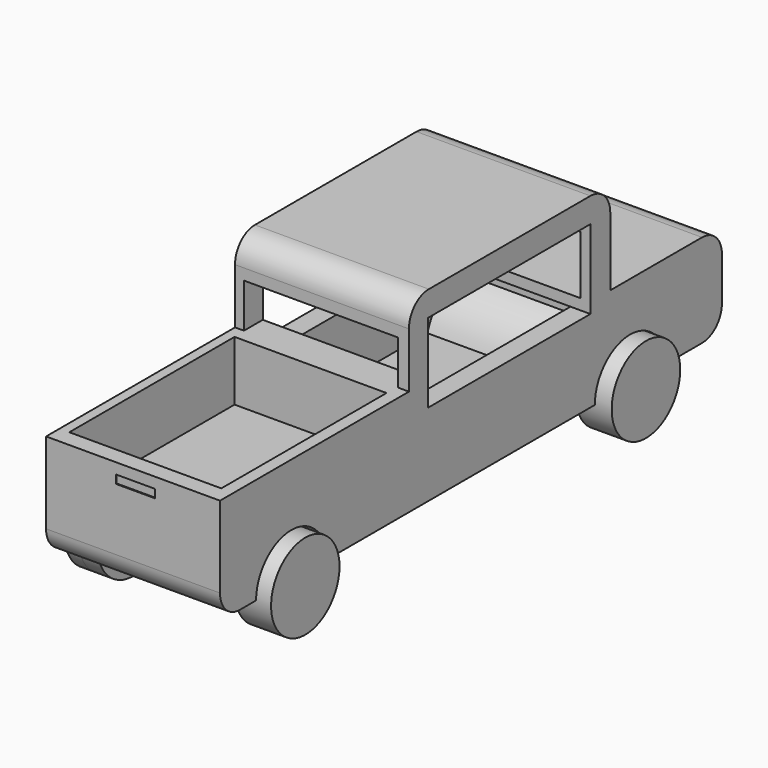
from build123d import *

# Parameters (mm, degrees)
F1_DEPTH      = 44.45
F3_DEPTH      = 46.99
F4_W          = 38.835483836
F4_H          = 52.7764223516
F5_DEPTH      = 15.24
F7_START      = 39.116
F6_R          = 10.9261370184
F7_DEPTH      = 9.144
F6_R_2        = 10.9431249162
F8_R          = 11.010831959
F9_DEPTH      = 3.556
F9_DEPTH_BACK = 4.826
F8_R_2        = 11.5864067576
F10_W         = 10.0583992898
F10_H         = 2.1336004138
F11_DEPTH     = 0.254
F12_W         = 51.9430035889
F12_H         = 20.2183979881
F13_DEPTH     = 55.118
F14_W         = 39.3191990443
F14_H         = 11.2776011229
F15_DEPTH     = 25.4
F16_T         = 5.08
F16_T3_DEPTH  = 54.61
F16_T5_DEPTH  = 12.4460015742
F16_T7_DEPTH  = 13.0047993815
F16_T9_DEPTH  = 16.1797990388
F16_T11_DEPTH = 25.4
F16_T13_DEPTH = 62.9364223516
F16_T15_DEPTH = 48.995483836
F16_T17_DEPTH = 10.414
F16_T19_DEPTH = 12.2936004138
F16_T21_DEPTH = 20.2183992898
F17_W         = 39.0143997502
F17_H         = 14.9351991713
F18_DEPTH     = 25.4


# Not quite as in the source:
# - a shell that OpenCascade refuses in one call is made with other operations: the cavity is built on its own and cut out


with BuildPart() as f1:
    # F0 (on Right) → F1 (new body)
    with BuildSketch(Plane.YZ):
        with BuildLine():
            Line((34.8995998502, 0), (34.8995998502, 23.7744003534))
            Line((34.8995998502, 23.7744003534), (34.8995998502, 41.2495988739))
            ThreePointArc((34.8995998502, 41.2495988739), (33.0397279107, 45.7397269344), (28.5495998502, 47.5995988739))
            Line((28.5495998502, 47.5995988739), (-23.0632027775, 47.5995988739))
            ThreePointArc((-23.0632027775, 47.5995988739), (-27.553330838, 45.7397269344), (-29.4132027775, 41.2495988739))
            Line((-29.4132027775, 41.2495988739), (-29.4132027775, 27.127198875))
            Line((-29.4132027775, 27.127198875), (-29.4132027775, 0))
            Line((-29.4132027775, 0), (34.8995998502, 0))
        make_face()
        with BuildLine():
            Line((-83.4136041045, 0), (-29.4132027775, 0))
            Line((-29.4132027775, 0), (-29.4132027775, 27.127198875))
            Line((-29.4132027775, 27.127198875), (-89.7636041045, 27.127198875))
            Line((-89.7636041045, 27.127198875), (-89.7636041045, 6.35))
            ThreePointArc((-89.7636041045, 6.35), (-87.9037321651, 1.8598719395), (-83.4136041045, 0))
        make_face()
        with BuildLine():
            Line((64.2112003803, 23.7744003534), (34.8995998502, 23.7744003534))
            Line((34.8995998502, 23.7744003534), (34.8995998502, 0))
            Line((34.8995998502, 0), (64.2112003803, 0))
            ThreePointArc((64.2112003803, 0), (68.7013284409, 1.8598719395), (70.5612003803, 6.35))
            Line((70.5612003803, 6.35), (70.5612003803, 17.4244003534))
            ThreePointArc((70.5612003803, 17.4244003534), (68.7013284409, 21.914528414), (64.2112003803, 23.7744003534))
        make_face()
    extrude(amount=F1_DEPTH)

    # F2 (on face) → F3 (cut)
    with BuildSketch(Plane.YZ.offset(44.45)):
        with BuildLine():
            ThreePointArc((52.4891002785, 0), (41.2242002785, 11.2649), (29.9593002785, 0))
            Line((29.9593002785, 0), (52.4891002785, 0))
        make_face()
        with BuildLine():
            Line((-78.2477574524, 0), (-55.7118488375, 0))
            ThreePointArc((-55.7118488375, 0), (-66.9798031449, 11.2679543074), (-78.2477574524, 0))
        make_face()
        with BuildLine():
            Line((52.4891002785, 0), (29.9593002785, 0))
            ThreePointArc((29.9593002785, 0), (41.2242002785, -11.2649), (52.4891002785, 0))
        make_face()
        with BuildLine():
            ThreePointArc((-78.2477574524, 0), (-66.9798031449, -11.2679543074), (-55.7118488375, 0))
            Line((-55.7118488375, 0), (-78.2477574524, 0))
        make_face()
    extrude(amount=-F3_DEPTH, mode=Mode.SUBTRACT)

    # F4 (on face) → F5 (cut)
    with BuildSketch(Plane.XY.offset(27.127198875)):
        with Locations((21.9071976608, -59.0603370219)):
            Rectangle(F4_W, F4_H)
    extrude(amount=-F5_DEPTH, mode=Mode.SUBTRACT)

    # F10 (on face) → F11 (cut)
    with BuildSketch(Plane.XZ.offset(89.7636041045)):
        with Locations((22.85999991, 23.317201063)):
            Rectangle(F10_W, F10_H)
    extrude(amount=-F11_DEPTH, mode=Mode.SUBTRACT)

    # F12 (on face) → F13 (cut)
    with BuildSketch(Plane(origin=(0, 0, 0), x_dir=(0, -1, 0), z_dir=(-1, 0, 0))):
        with Locations((-2.5780980557, 31.1403998798)):
            Rectangle(F12_W, F12_H)
    extrude(amount=-F13_DEPTH, mode=Mode.SUBTRACT)

    # F14 (on face) → F15 (cut)
    with BuildSketch(Plane.XZ.offset(29.4132027775)):
        with Locations((21.9456010964, 32.7659994364)):
            Rectangle(F14_W, F14_H)
    extrude(amount=-F15_DEPTH, mode=Mode.SUBTRACT)

    # F16: shell of thickness 5.08, made by hand


with BuildPart() as f7:
    # F6 (on Right) → F7 (new body)
    with BuildSketch(Plane.YZ.offset(F7_START)):
        with Locations((-67.2845989466, 0)):
            Circle(F6_R)
    extrude(amount=F7_DEPTH)


with BuildPart() as f7b:
    # F6 (on Right) → F7, piece 2 (new body)
    with BuildSketch(Plane.YZ.offset(F7_START)):
        with Locations((41.5289998055, 0)):
            Circle(F6_R_2)
    extrude(amount=F7_DEPTH)


with BuildPart() as f9:
    # F8 (on Right) → F9 (new body, two sides)
    with BuildSketch(Plane.YZ) as f9_sk:
        with Locations((41.8337993324, 0)):
            Circle(F8_R)
    extrude(amount=-F9_DEPTH)
    extrude(f9_sk.sketch, amount=F9_DEPTH_BACK)


with BuildPart() as f9b:
    # F8 (on Right) → F9, piece 2 (new body, two sides)
    with BuildSketch(Plane.YZ) as f9_2_sk:
        with Locations((-67.8941980004, 0)):
            Circle(F8_R_2)
    extrude(amount=-F9_DEPTH)
    extrude(f9_2_sk.sketch, amount=F9_DEPTH_BACK)


with BuildPart() as f16_core1:
    # F16_t2: copy of F1
    add(f1.part)

    # the walls: a layer under each face that stays
    f16_faces = [f16_core1.faces().sort_by_distance(p)[0] for p in [
        (22.225, 34.8995998502, 32.5119996136),
        (22.225, 49.5554001153, 23.7744003534),
        (22.225, 33.0397279107, 45.7397269344),
        (0, -63.042803357, 23.7997994369),
        (44.45, -63.042803357, 23.7997994369),
        (22.225, 68.7013284409, 21.914528414),
        (22.225, 2.7431985363, 47.5995988739),
        (22.225, 70.5612003803, 11.8872001767),
        (22.225, 68.7013284409, 1.8598719395),
        (22.225, 58.3501503294, 0),
        (22.225, -27.553330838, 45.7397269344),
        (22.225, 41.2242002785, 11.2649),
        (37.0416666667, -29.4132027775, 38.8958655407),
        (22.225, -12.8762742795, 0),
        (41.275, -28.1341323363, 27.127198875),
        (22.225, -66.9798031449, 11.2679543074),
        (22.225, -89.7636041045, 16.7385994375),
        (22.225, -80.8306807784, 0),
        (22.225, -87.9037321651, 1.8598719395),
        (22.225, 28.5495998502, 31.1403998798),
        (22.225, 2.5780980557, 41.2495988739),
        (37.0416666667, -23.3934037387, 24.4009338838),
        (2.2860015742, -26.4033032581, 32.7659994364),
        (21.9456010964, -26.4033032581, 38.4047999978),
        (41.6052006185, -26.4033032581, 32.7659994364),
        (41.3249395788, -59.0603370219, 19.507198875),
        (21.9071976608, -85.4485481977, 19.507198875),
        (2.4894557428, -59.0603370219, 19.507198875),
        (21.9071976608, -32.6721258461, 19.507198875),
        (27.8891995549, -89.6366041045, 23.317201063),
        (22.85999991, -89.6366041045, 22.2504008561),
        (17.8308002651, -89.6366041045, 23.317201063),
        (22.85999991, -89.6366041045, 24.3840012699),
        (21.9071976608, -59.0603370219, 11.887198875),
        (22.85999991, -89.5096041045, 23.317201063),
    ]]
    thicken(f16_faces, amount=-F16_T, mode=Mode.SUBTRACT)

    # F16_s4 → F16_t3 (cut)
    with BuildSketch(Plane.YZ.offset(-5.08)):
        Polygon((34.9503998502, 23.8252003534), (29.8195998502, 23.7744003534), (29.8195998502, 18.6944003534), (34.8995998502, 18.6944003534), align=None)
        Polygon((28.4987998502, 41.1987988739), (33.6295998502, 41.2495988739), (33.6295998502, 46.3295988739), (28.5495998502, 46.3295988739), align=None)
        Polygon((-23.3426037387, 41.1987988739), (-23.3934037387, 46.3295988739), (-28.4734037387, 46.3295988739), (-28.4734037387, 41.2495988739), align=None)
    extrude(amount=F16_T3_DEPTH, mode=Mode.SUBTRACT)

    # F16_s6 → F16_t5 (cut)
    with BuildSketch(Plane.YZ.offset(-5.08)):
        Polygon((-29.4640027775, 27.177998875), (-24.3332027775, 27.127198875), (-24.3332027775, 22.047198875), (-29.4132027775, 22.047198875), align=None)
    extrude(amount=F16_T5_DEPTH, mode=Mode.SUBTRACT)

    # F16_s8 → F16_t7 (cut)
    with BuildSketch(Plane.YZ.offset(36.5252006185)):
        Polygon((-29.4640027775, 27.177998875), (-24.3332027775, 27.127198875), (-24.3332027775, 22.047198875), (-29.4132027775, 22.047198875), align=None)
    extrude(amount=F16_T7_DEPTH, mode=Mode.SUBTRACT)

    # F16_s10 → F16_t9 (cut)
    with BuildSketch(Plane.XZ.offset(18.3134037387)):
        Polygon((2.3368015742, 27.177998875), (2.2860015742, 22.047198875), (-2.7939984258, 22.047198875), (-2.7939984258, 27.127198875), align=None)
        Polygon((41.5544006185, 27.177998875), (41.6052006185, 22.047198875), (46.6852006185, 22.047198875), (46.6852006185, 27.127198875), align=None)
        Polygon((2.3368015742, 38.3539999978), (-2.7939984258, 38.4047999978), (-2.7939984258, 43.4847999978), (2.2860015742, 43.4847999978), align=None)
        Polygon((41.5544006185, 38.3539999978), (41.6052006185, 43.4847999978), (46.6852006185, 43.4847999978), (46.6852006185, 38.4047999978), align=None)
    extrude(amount=F16_T9_DEPTH, mode=Mode.SUBTRACT)

    # F16_s12 → F16_t11 (cut)
    with BuildSketch(Plane.XY.offset(6.807198875)):
        Polygon((41.2741395788, -85.3977481977), (46.4049395788, -85.4485481977), (46.4049395788, -90.5285481977), (41.3249395788, -90.5285481977), align=None)
        Polygon((41.2741395788, -32.7229258461), (46.4049395788, -32.6721258461), (46.4049395788, -27.5921258461), (41.3249395788, -27.5921258461), align=None)
        Polygon((2.5402557428, -85.3977481977), (2.4894557428, -90.5285481977), (-2.5905442572, -90.5285481977), (-2.5905442572, -85.4485481977), align=None)
        Polygon((2.5402557428, -32.7229258461), (-2.5905442572, -32.6721258461), (-2.5905442572, -27.5921258461), (2.4894557428, -27.5921258461), align=None)
    extrude(amount=F16_T11_DEPTH, mode=Mode.SUBTRACT)

    # F16_s14 → F16_t13 (cut)
    with BuildSketch(Plane.XZ.offset(27.5921258461)):
        Polygon((41.2741395788, 11.937998875), (46.4049395788, 11.887198875), (46.4049395788, 6.807198875), (41.3249395788, 6.807198875), align=None)
        Polygon((2.5402557428, 11.937998875), (-2.5905442572, 11.887198875), (-2.5905442572, 6.807198875), (2.4894557428, 6.807198875), align=None)
    extrude(amount=F16_T13_DEPTH, mode=Mode.SUBTRACT)

    # F16_s16 → F16_t15 (cut)
    with BuildSketch(Plane.YZ.offset(-2.5905442572)):
        Polygon((-85.3977481977, 11.937998875), (-90.5285481977, 11.887198875), (-90.5285481977, 6.807198875), (-85.4485481977, 6.807198875), align=None)
        Polygon((-32.7229258461, 11.937998875), (-27.5921258461, 11.887198875), (-27.5921258461, 6.807198875), (-32.6721258461, 6.807198875), align=None)
    extrude(amount=F16_T15_DEPTH, mode=Mode.SUBTRACT)

    # F16_s18 → F16_t17 (cut)
    with BuildSketch(Plane.XZ.offset(84.4296041045)):
        Polygon((27.8383995549, 22.3012008561), (32.9691995549, 22.2504008561), (32.9691995549, 17.1704008561), (27.8891995549, 17.1704008561), align=None)
        Polygon((27.8383995549, 24.3332012699), (32.9691995549, 24.3840012699), (32.9691995549, 29.4640012699), (27.8891995549, 29.4640012699), align=None)
        Polygon((17.8816002651, 22.3012008561), (17.8308002651, 17.1704008561), (12.7508002651, 17.1704008561), (12.7508002651, 22.2504008561), align=None)
        Polygon((17.8816002651, 24.3332012699), (12.7508002651, 24.3840012699), (12.7508002651, 29.4640012699), (17.8308002651, 29.4640012699), align=None)
    extrude(amount=F16_T17_DEPTH, mode=Mode.SUBTRACT)

    # F16_s20 → F16_t19 (cut)
    with BuildSketch(Plane.XY.offset(17.1704008561)):
        Polygon((27.8383995549, -89.5604041045), (32.9691995549, -89.5096041045), (32.9691995549, -84.4296041045), (27.8891995549, -84.4296041045), align=None)
        Polygon((17.8816002651, -89.5604041045), (12.7508002651, -89.5096041045), (12.7508002651, -84.4296041045), (17.8308002651, -84.4296041045), align=None)
    extrude(amount=F16_T19_DEPTH, mode=Mode.SUBTRACT)

    # F16_s22 → F16_t21 (cut)
    with BuildSketch(Plane.YZ.offset(12.7508002651)):
        Polygon((-89.5604041045, 22.3012008561), (-89.5096041045, 17.1704008561), (-84.4296041045, 17.1704008561), (-84.4296041045, 22.2504008561), align=None)
        Polygon((-89.5604041045, 24.3332012699), (-89.5096041045, 29.4640012699), (-84.4296041045, 29.4640012699), (-84.4296041045, 24.3840012699), align=None)
    extrude(amount=F16_T21_DEPTH, mode=Mode.SUBTRACT)


with BuildPart() as f1_1:
    add(f1.part)

    # what is left inside the walls is the cavity
    f16_cavity = [f16_core1.part.solids().sort_by_distance(p)[0] for p in [
        (27.94, -12.876195, 5.1308),
        (22.225, -83.73677, 6.756399),
    ]]
    add(f16_cavity, mode=Mode.SUBTRACT)

    # F17 (on face) → F18 (cut)
    with BuildSketch(Plane(origin=(0, 34.8995998502, 0), x_dir=(-1, 0, 0), z_dir=(0, 1, 0))):
        with Locations((-22.4028002704, 31.2419999391)):
            Rectangle(F17_W, F17_H)
    extrude(amount=-F18_DEPTH, mode=Mode.SUBTRACT)


solid = Compound([f7.part, f7b.part, f9.part, f9b.part, f1_1.part])
